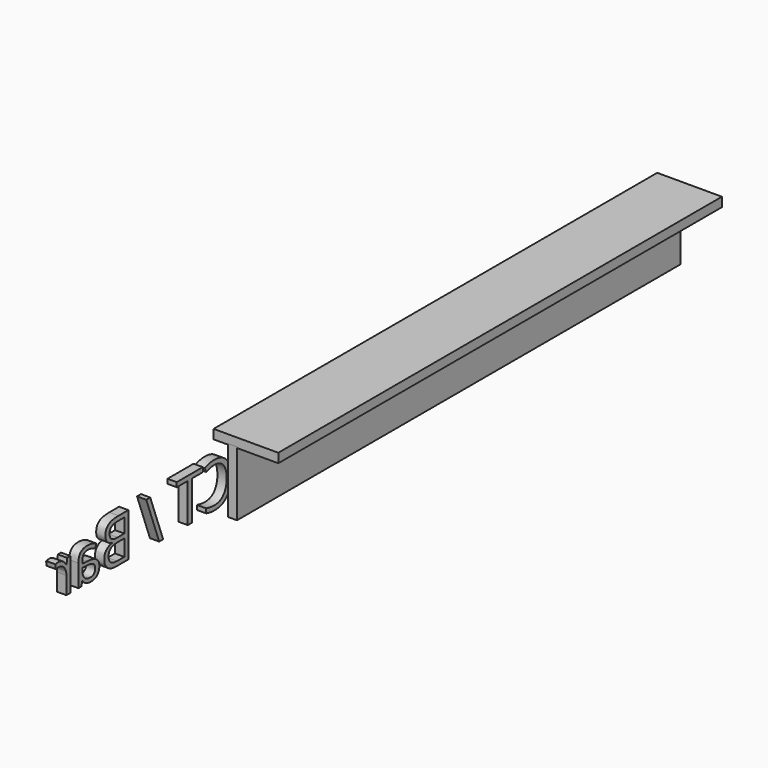
from build123d import *

# Parameters (mm, degrees)
F0_W         = 100
F0_H         = 700
F1_DEPTH     = 6000
F3_DEPTH     = 6000
F4_TEXT_SIZE = 658.3185866475
F5_DEPTH     = 100


# Not quite as in the source:
# - Text() gives the source's letters only with a copy of the font that has no kerning and outlines rounded to 1/6400 em; it was checked with that copy


with BuildPart() as f1:
    # F0 (on Front) → F1 (new body)
    with BuildSketch(Plane.XZ):
        Rectangle(F0_W, F0_H)
    extrude(amount=F1_DEPTH)


with BuildPart() as f3:
    # F2 (on face) → F3 (new body)
    with BuildSketch(Plane.XZ.offset(6000)):
        Polygon((-203.4594625484, 438.7127488852), (-203.4594625484, 338.7127488852), (-50, 338.7127488852), (-50, 350), (50, 350), (50, 338.7127488852), (496.5405374516, 338.7127488852), (496.5405374516, 349.2390767514), (496.5405374516, 438.7127488852), align=None)
    extrude(amount=-F3_DEPTH)


with BuildPart() as f5:
    # F4 (on face) → F5 (new body)
    with BuildSketch(Plane(origin=(-50, 0, 0), x_dir=(0, -1, 0), z_dir=(-1, 0, 0))):
        with Locations((119.3822026253, -208.4814757109)):
            Text('Reception / Shop / CT / Bar', F4_TEXT_SIZE, font='Open Sans', text_align=(TextAlign.LEFT, TextAlign.BOTTOM))
    extrude(amount=F5_DEPTH)


solid = Compound([f1.part, f3.part, f5.part])
